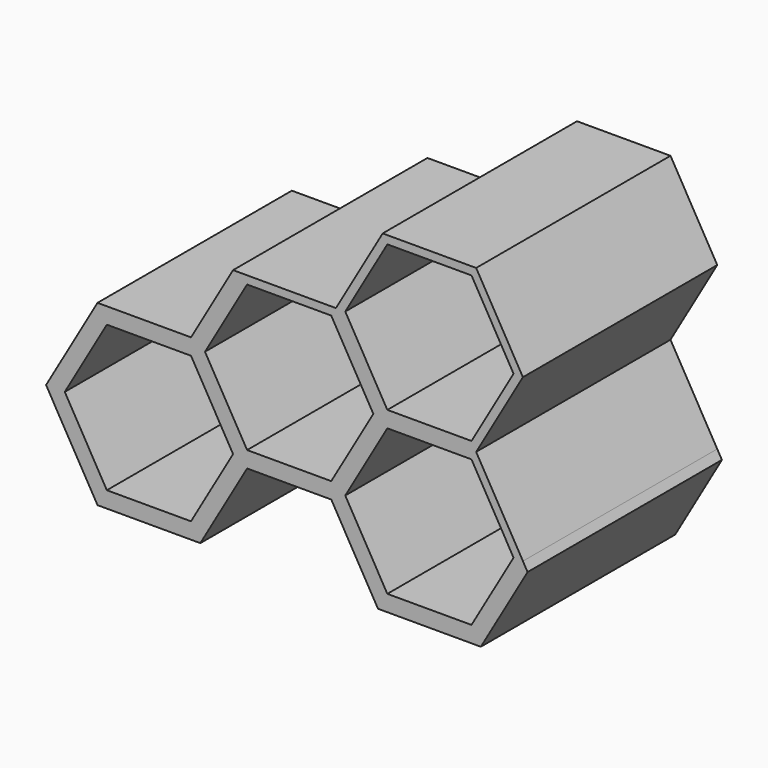
from build123d import *

# Parameters (mm, degrees)
F1_DEPTH = 12.7
F2_DEPTH = 95.25


# Not quite as in the source:
# - a feature names something its author has since deleted; it is built from what else it names


with BuildPart() as f1:
    # F0 (on Front) → F1 (new body)
    with BuildSketch(Plane.XZ):
        Polygon((-187.5869779497, -91.9575006988), (-169.2561069029, -60.2075006988), (-187.5869779497, -28.4575006988), (-224.2487200432, -28.4575006988), (-242.57959109, -60.2075006988), (-224.2487200432, -91.9575006988), align=None)
        Polygon((-222.4156329385, -88.7825006988), (-238.9134168806, -60.2075006988), (-222.4156329385, -31.6325006988), (-189.4200650544, -31.6325006988), (-172.9222811123, -60.2075006988), (-189.4200650544, -88.7825006988), align=None, mode=Mode.SUBTRACT)
        Polygon((-59.2708806223, -60.2075006988), (-77.6017516691, -28.4575006988), (-114.2634937626, -28.4575006988), (-132.5943648094, -60.2075006988), (-114.2634937626, -91.9575006988), (-77.6017516691, -91.9575006988), align=None)
        Polygon((-112.4304066579, -88.7825006988), (-128.9281906, -60.2075006988), (-112.4304066579, -31.6325006988), (-79.4348387737, -31.6325006988), (-62.9370548316, -60.2075006988), (-79.4348387737, -88.7825006988), align=None, mode=Mode.SUBTRACT)
        Polygon((-77.6017516691, -28.4575006988), (-59.2708806223, 3.2924993012), (-77.6017516691, 35.0424993012), (-114.2634937626, 35.0424993012), (-132.5943648094, 3.2924993012), (-114.2634937626, -28.4575006988), align=None)
        Polygon((-112.4304066579, -25.2825006988), (-128.9281906, 3.2924993012), (-112.4304066579, 31.8674993012), (-79.4348387737, 31.8674993012), (-62.9370548316, 3.2924993012), (-79.4348387737, -25.2825006988), align=None, mode=Mode.SUBTRACT)
        Polygon((-132.5943648094, -60.2075006988), (-114.2634937626, -28.4575006988), (-132.5943648094, 3.2924993012), (-169.2561069029, 3.2924993012), (-187.5869779497, -28.4575006988), (-169.2561069029, -60.2075006988), align=None)
        Polygon((-167.4230197982, -57.0325006988), (-183.9208037403, -28.4575006988), (-167.4230197982, 0.1174993012), (-134.4274519141, 0.1174993012), (-117.929667972, -28.4575006988), (-134.4274519141, -57.0325006988), align=None, mode=Mode.SUBTRACT)
        Polygon((-222.4156329385, -31.6325006988), (-238.9134168806, -60.2075006988), (-222.4156329385, -88.7825006988), (-189.4200650544, -88.7825006988), (-172.9222811123, -60.2075006988), (-189.4200650544, -31.6325006988), align=None)
        Polygon((-112.4304066579, -31.6325006988), (-128.9281906, -60.2075006988), (-112.4304066579, -88.7825006988), (-79.4348387737, -88.7825006988), (-62.9370548316, -60.2075006988), (-79.4348387737, -31.6325006988), align=None)
        Polygon((-167.4230197982, 0.1174993012), (-183.9208037403, -28.4575006988), (-167.4230197982, -57.0325006988), (-134.4274519141, -57.0325006988), (-117.929667972, -28.4575006988), (-134.4274519141, 0.1174993012), align=None)
        Polygon((-112.4304066579, 31.8674993012), (-128.9281906, 3.2924993012), (-112.4304066579, -25.2825006988), (-79.4348387737, -25.2825006988), (-62.9370548316, 3.2924993012), (-79.4348387737, 31.8674993012), align=None)
    extrude(amount=F1_DEPTH)

    # F0 (on Front) → F2 (join)
    with BuildSketch(Plane.XZ):
        Polygon((-77.6017516691, -28.4575006988), (-59.2708806223, 3.2924993012), (-77.6017516691, 35.0424993012), (-114.2634937626, 35.0424993012), (-132.5943648094, 3.2924993012), (-114.2634937626, -28.4575006988), align=None)
        Polygon((-112.4304066579, -25.2825006988), (-128.9281906, 3.2924993012), (-112.4304066579, 31.8674993012), (-79.4348387737, 31.8674993012), (-62.9370548316, 3.2924993012), (-79.4348387737, -25.2825006988), align=None, mode=Mode.SUBTRACT)
        Polygon((-59.2708806223, -60.2075006988), (-77.6017516691, -28.4575006988), (-114.2634937626, -28.4575006988), (-132.5943648094, -60.2075006988), (-114.2634937626, -91.9575006988), (-77.6017516691, -91.9575006988), align=None)
        Polygon((-112.4304066579, -88.7825006988), (-128.9281906, -60.2075006988), (-112.4304066579, -31.6325006988), (-79.4348387737, -31.6325006988), (-62.9370548316, -60.2075006988), (-79.4348387737, -88.7825006988), align=None, mode=Mode.SUBTRACT)
        Polygon((-132.5943648094, -60.2075006988), (-114.2634937626, -28.4575006988), (-132.5943648094, 3.2924993012), (-169.2561069029, 3.2924993012), (-187.5869779497, -28.4575006988), (-169.2561069029, -60.2075006988), align=None)
        Polygon((-167.4230197982, -57.0325006988), (-183.9208037403, -28.4575006988), (-167.4230197982, 0.1174993012), (-134.4274519141, 0.1174993012), (-117.929667972, -28.4575006988), (-134.4274519141, -57.0325006988), align=None, mode=Mode.SUBTRACT)
        Polygon((-187.5869779497, -91.9575006988), (-169.2561069029, -60.2075006988), (-187.5869779497, -28.4575006988), (-224.2487200432, -28.4575006988), (-242.57959109, -60.2075006988), (-224.2487200432, -91.9575006988), align=None)
        Polygon((-222.4156329385, -88.7825006988), (-238.9134168806, -60.2075006988), (-222.4156329385, -31.6325006988), (-189.4200650544, -31.6325006988), (-172.9222811123, -60.2075006988), (-189.4200650544, -88.7825006988), align=None, mode=Mode.SUBTRACT)
        Polygon((-57.4378374826, -63.3825006988), (-59.2708806223, -60.2075006988), (-77.6017516691, -91.9575006988), (-114.2634937626, -91.9575006988), (-132.5943648094, -60.2075006988), (-169.2561069029, -60.2075006988), (-187.5869779497, -91.9575006988), (-224.2487200432, -91.9575006988), (-242.57959109, -60.2075006988), (-224.2487200432, -28.4575006988), (-187.5869779497, -28.4575006988), (-169.2561069029, 3.2924993012), (-172.9222811123, 3.2924993012), (-189.4200540638, -25.2824816625), (-226.0817961573, -25.2824816625), (-246.24577629, -60.2075197352), (-226.0817961573, -95.1325578078), (-185.7539677819, -95.1325578078), (-167.4230967351, -63.3825578078), (-134.4273749772, -63.3825578078), (-116.0965039304, -95.1325578078), (-75.7687415012, -95.1325578078), align=None)
    extrude(amount=F2_DEPTH)


solid = f1.part
